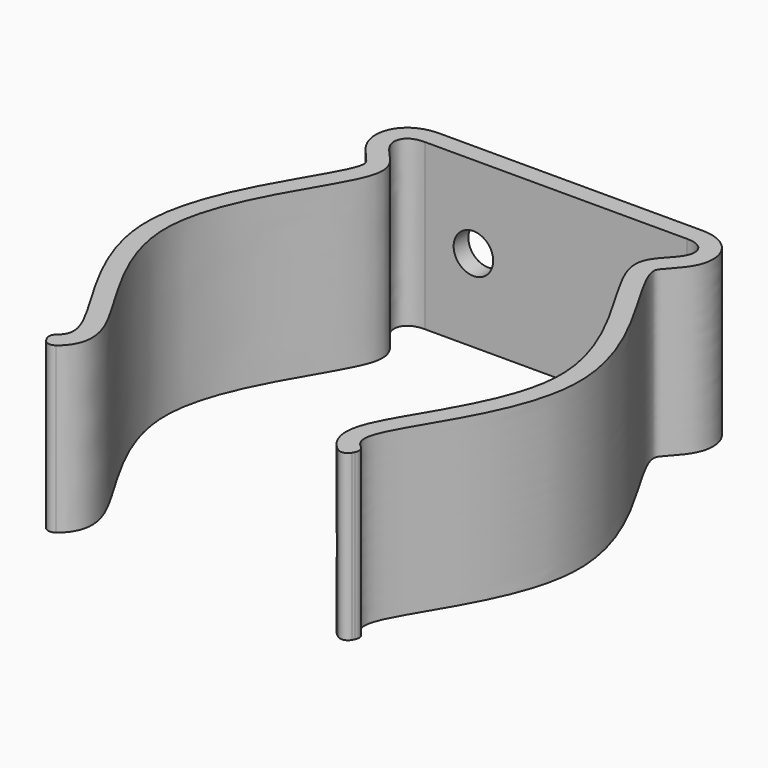
from build123d import *

# Parameters (mm, degrees)
F1_DEPTH = 25
F2_R     = 3
F3_DEPTH = 25
F4_R     = 1.2


# Not quite as in the source:
# - the dataset's text gives a spline's control points without its knots; the knots are read off the source's solid


with BuildPart() as f1:
    # F0 (on Top) → F1 (new body)
    with BuildSketch(Plane.XY):
        with BuildLine():
            Line((-19.8750495911, 0), (0, 0))
            Line((0, 0), (19.8750495911, 0))
            add(Edge.make_bspline(
                [(19.8750495911, 0), (22.2924524796, -9.5208e-06), (23.8468038816, -3.0523168549), (19.0693924552, -6.5670221707), (18.6729332639, -12.7588770638), (37.9576470343, -36.8571689193), (18.3568969249, -59.7122156399), (19.423014069, -66.4084536548), (21.2647124099, -68.0696110384), (22.562418133, -68.7783882022)],
                knots=[0, 0, 0, 0, 0.0945411672, 0.1993686999, 0.3071885555, 0.5544117499, 0.7986209568, 0.9087635251, 1, 1, 1, 1], degree=3))
            Line((22.562418133, -68.7783882022), (23.9045723519, -66.3210274121))
            add(Edge.make_bspline(
                [(19.8750606187, 2.8), (20.4593069859, 2.799997699), (21.5883647785, 2.6863173566), (22.9032546448, 2.1968633988), (23.8314426543, 1.5684869445), (24.435854505, 0.9880902727), (24.9232939323, 0.3201474741), (25.2783951523, -0.4034584687), (25.4999568914, -1.1503426565), (25.5971545038, -1.8950756512), (25.5834825611, -2.6207983738), (25.4901886128, -3.2034968646), (25.3716356249, -3.6511053376), (25.2309586179, -4.0723173675), (25.0214545116, -4.5538263985), (24.7391708776, -5.0639453956), (24.3421099364, -5.6682154891), (23.8341446747, -6.3080287414), (23.2580066814, -6.9526509281), (22.8386460714, -7.410690486), (22.5605388052, -7.729409075), (22.3860591598, -7.9412155998), (22.2498645667, -8.1219170001), (22.1266426007, -8.3070114205), (22.0377754259, -8.4824771505), (21.9903206529, -8.6321382793), (21.9643998721, -8.8002455288), (21.9686979601, -9.0763133266), (22.0440959051, -9.5144686085), (22.2308250058, -10.1312073308), (22.5534171189, -10.9208744064), (23.0327923343, -11.902651775), (23.8450711076, -13.4119164755), (25.1238572248, -15.6160909141), (26.8903289815, -18.6544793295), (28.7108310762, -22.0166637858), (30.4105304557, -25.6498365655), (31.5779576864, -28.871182811), (32.2660810741, -31.5495260763), (32.6319090351, -33.6054292675), (32.8205512079, -35.7013715538), (32.794715562, -37.8351090141), (32.5567271095, -39.9175968775), (32.0063619416, -42.6269799256), (30.952903282, -45.8715528951), (29.318855882, -49.5212306518), (27.5054488177, -52.9067151854), (25.696037368, -55.9942070619), (24.3447227252, -58.2762559642), (23.4533034554, -59.8831067643), (22.904028849, -60.9607111118), (22.5664151147, -61.7287262628), (22.3761997694, -62.2470363726), (22.2269924721, -62.7232034294), (22.1127869942, -63.2322655125), (22.0628810378, -63.7177729426), (22.0729996001, -64.0971510525), (22.1220907308, -64.4007199093), (22.1879270254, -64.6196927194), (22.2568363773, -64.7893256597), (22.317850339, -64.9168005859), (22.3885249864, -65.0451322219), (22.4837806609, -65.1967051299), (22.61356875, -65.3686320853), (22.8083966888, -65.5738545979), (23.1579171235, -65.8716332359), (23.5589591357, -66.1322613839), (23.9045723519, -66.3210274121)],
                knots=[0, 0, 0, 0, 0.015625, 0.03125, 0.0390625, 0.046875, 0.0546875, 0.0625, 0.0703125, 0.078125, 0.0859375, 0.09375, 0.09765625, 0.1015625, 0.109375, 0.1171875, 0.125, 0.140625, 0.15625, 0.171875, 0.1796875, 0.1875, 0.1953125, 0.203125, 0.21875, 0.234375, 0.25, 0.265625, 0.28125, 0.296875, 0.3125, 0.328125, 0.34375, 0.375, 0.40625, 0.4375, 0.46875, 0.5, 0.515625, 0.53125, 0.546875, 0.5625, 0.578125, 0.59375, 0.625, 0.65625, 0.6875, 0.71875, 0.75, 0.765625, 0.78125, 0.796875, 0.8046875, 0.8125, 0.828125, 0.84375, 0.859375, 0.875, 0.890625, 0.8984375, 0.90625, 0.9140625, 0.921875, 0.9375, 0.953125, 0.96875, 1, 1, 1, 1], degree=3))
            Line((19.8750606187, 2.8), (0, 2.8))
            Line((0, 2.8), (-19.8750606187, 2.8))
            add(Edge.make_bspline(
                [(-19.8750606187, 2.8), (-20.4593069859, 2.799997699), (-21.5883647785, 2.6863173566), (-22.9032546448, 2.1968633988), (-23.8314426543, 1.5684869445), (-24.435854505, 0.9880902727), (-24.9232939323, 0.3201474741), (-25.2783951523, -0.4034584687), (-25.4999568914, -1.1503426565), (-25.5971545038, -1.8950756512), (-25.5834825611, -2.6207983738), (-25.4901886128, -3.2034968646), (-25.3716356249, -3.6511053376), (-25.2309586179, -4.0723173675), (-25.0214545116, -4.5538263985), (-24.7391708776, -5.0639453956), (-24.3421099364, -5.6682154891), (-23.8341446747, -6.3080287414), (-23.2580066814, -6.9526509281), (-22.8386460714, -7.410690486), (-22.5605388052, -7.729409075), (-22.3860591598, -7.9412155998), (-22.2498645667, -8.1219170001), (-22.1266426007, -8.3070114205), (-22.0377754259, -8.4824771505), (-21.9903206529, -8.6321382793), (-21.9643998721, -8.8002455288), (-21.9686979601, -9.0763133266), (-22.0440959051, -9.5144686085), (-22.2308250058, -10.1312073308), (-22.5534171189, -10.9208744064), (-23.0327923343, -11.902651775), (-23.8450711076, -13.4119164755), (-25.1238572248, -15.6160909141), (-26.8903289815, -18.6544793295), (-28.7108310762, -22.0166637858), (-30.4105304557, -25.6498365655), (-31.5779576864, -28.871182811), (-32.2660810741, -31.5495260763), (-32.6319090351, -33.6054292675), (-32.8205512079, -35.7013715538), (-32.794715562, -37.8351090141), (-32.5567271095, -39.9175968775), (-32.0063619416, -42.6269799256), (-30.952903282, -45.8715528951), (-29.318855882, -49.5212306518), (-27.5054488177, -52.9067151854), (-25.696037368, -55.9942070619), (-24.3447227252, -58.2762559642), (-23.4533034554, -59.8831067643), (-22.904028849, -60.9607111118), (-22.5664151147, -61.7287262628), (-22.3761997694, -62.2470363726), (-22.2269924721, -62.7232034294), (-22.1127869942, -63.2322655125), (-22.0628810378, -63.7177729426), (-22.0729996001, -64.0971510525), (-22.1220907308, -64.4007199093), (-22.1879270254, -64.6196927194), (-22.2568363773, -64.7893256597), (-22.317850339, -64.9168005859), (-22.3885249864, -65.0451322219), (-22.4837806609, -65.1967051299), (-22.61356875, -65.3686320853), (-22.8083966888, -65.5738545979), (-23.1579171235, -65.8716332359), (-23.5589591357, -66.1322613839), (-23.9045723519, -66.3210274121)],
                knots=[0, 0, 0, 0, 0.015625, 0.03125, 0.0390625, 0.046875, 0.0546875, 0.0625, 0.0703125, 0.078125, 0.0859375, 0.09375, 0.09765625, 0.1015625, 0.109375, 0.1171875, 0.125, 0.140625, 0.15625, 0.171875, 0.1796875, 0.1875, 0.1953125, 0.203125, 0.21875, 0.234375, 0.25, 0.265625, 0.28125, 0.296875, 0.3125, 0.328125, 0.34375, 0.375, 0.40625, 0.4375, 0.46875, 0.5, 0.515625, 0.53125, 0.546875, 0.5625, 0.578125, 0.59375, 0.625, 0.65625, 0.6875, 0.71875, 0.75, 0.765625, 0.78125, 0.796875, 0.8046875, 0.8125, 0.828125, 0.84375, 0.859375, 0.875, 0.890625, 0.8984375, 0.90625, 0.9140625, 0.921875, 0.9375, 0.953125, 0.96875, 1, 1, 1, 1], degree=3))
            Line((-23.9045723519, -66.3210274121), (-22.562418133, -68.7783882022))
            add(Edge.make_bspline(
                [(-19.8750495911, 0), (-22.2924524796, -9.5208e-06), (-23.8468038816, -3.0523168549), (-19.0693924552, -6.5670221707), (-18.6729332639, -12.7588770638), (-37.9576470343, -36.8571689193), (-18.3568969249, -59.7122156399), (-19.423014069, -66.4084536548), (-21.2647124099, -68.0696110384), (-22.562418133, -68.7783882022)],
                knots=[0, 0, 0, 0, 0.0945411672, 0.1993686999, 0.3071885555, 0.5544117499, 0.7986209568, 0.9087635251, 1, 1, 1, 1], degree=3))
        make_face()
    extrude(amount=F1_DEPTH)

    # F2 (on face) → F3 (cut)
    with BuildSketch(Plane.XZ):
        with Locations((-12.5, 12.5)):
            Circle(F2_R)
        with Locations((12.5, 12.5)):
            Circle(F2_R)
    extrude(amount=-F3_DEPTH, mode=Mode.SUBTRACT)

    # F4
    f4_edges = [f1.edges().sort_by_distance(p)[0] for p in [
        (-22.562418, -68.778388, 12.5),
        (-23.904572, -66.321027, 12.5),
        (22.562418, -68.778388, 12.5),
        (23.904572, -66.321027, 12.5),
    ]]
    fillet(f4_edges, radius=F4_R)


solid = f1.part
